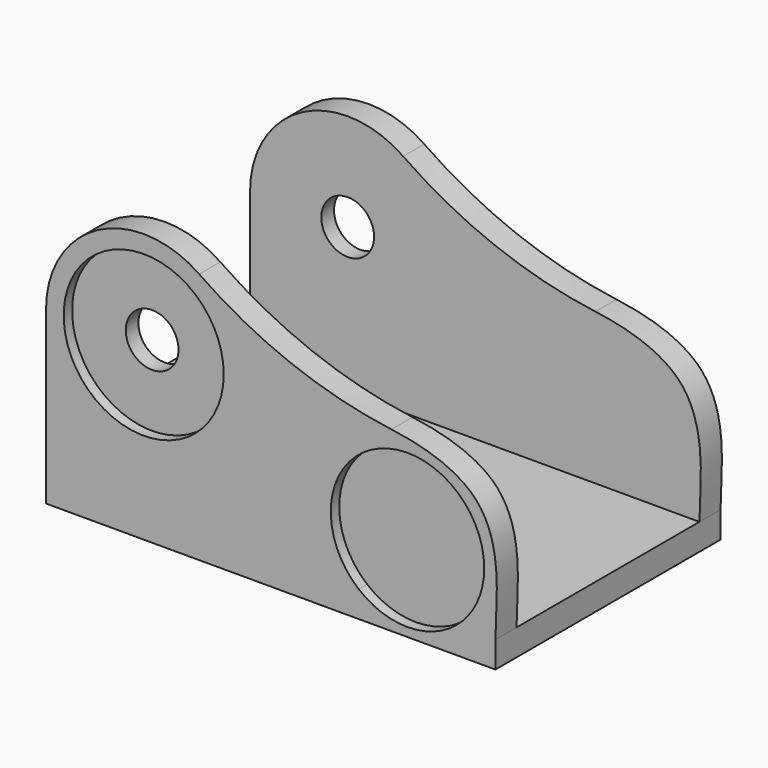
from build123d import *

# Parameters (mm, degrees)
F0_R            = 9.1
F0_W            = 2
F0_H            = 4
F0_R_2          = 3
F1_DEPTH        = 3
F1_COPIES_COUNT = 2
F1_COPIES_PITCH = 29
F2_DEPTH        = 32
F3_R            = 9.1
F4_DEPTH        = 3
F5_DEPTH        = 1.2
F3_R_2          = 3
F6_DEPTH        = 1.2


# Not quite as in the source:
# - a pattern or mirror of a feature is missing from the dataset's text; its kind, count and spacing are read off the source's solid


with BuildPart() as f1:
    # F0 (on Front) → F1 (new body)
    with BuildSketch(Plane.XZ):
        with BuildLine():
            Line((46.6587768439, 3), (51.1, 3))
            add(Edge.make_bspline(
                [(39.2721801194, 20.2002895195), (43.2600263156, 19.672514392), (52.7768717224, 16.5297183629), (51.1, 6.6124380804), (51.1, 3)],
                knots=[0.3415991708, 0.3415991708, 0.3415991708, 0.3415991708, 0.5830024084, 1, 1, 1, 1], degree=3))
            ThreePointArc((39.2721801194, 20.2002895195), (27.8400722418, 23.1174494268), (17.4097910893, 28.6321704107))
            ThreePointArc((17.4097910893, 28.6321704107), (5.9438716604, 29.329768082), (0, 19.5))
            Line((0, 19.5), (0, 7))
            Line((0, 7), (2, 7))
            Line((2, 7), (2, 3))
            Line((2, 3), (35.5412231561, 3))
            ThreePointArc((35.5412231561, 3), (37.3834628323, 17.6188568825), (49.825, 9.725))
            ThreePointArc((49.825, 9.725), (48.9938568825, 6.0084628323), (46.6587768439, 3))
        make_face()
        with Locations((11.1, 19.5)):
            Circle(F0_R, mode=Mode.SUBTRACT)
        with Locations((1, 5)):
            Rectangle(F0_W, F0_H)
        with BuildLine():
            Line((0, 3), (0, 0))
            Line((0, 0), (51.1, 0))
            Line((51.1, 0), (51.1, 3))
            Line((51.1, 3), (46.6587768439, 3))
            ThreePointArc((46.6587768439, 3), (41.1, 1), (35.5412231561, 3))
            Line((35.5412231561, 3), (2, 3))
            Line((2, 3), (0, 3))
        make_face()
        with BuildLine():
            Line((35.5412231561, 3), (46.6587768439, 3))
            ThreePointArc((46.6587768439, 3), (48.9938568825, 6.0084628323), (49.825, 9.725))
            ThreePointArc((49.825, 9.725), (37.3834628323, 17.6188568825), (35.5412231561, 3))
        make_face()
        with BuildLine():
            ThreePointArc((35.5412231561, 3), (41.1, 1), (46.6587768439, 3))
            Line((46.6587768439, 3), (35.5412231561, 3))
        make_face()
        with Locations((11.1, 19.5)):
            Circle(F0_R)
        with Locations((11.1, 19.5)):
            Circle(F0_R_2, mode=Mode.SUBTRACT)
    extrude(amount=-F1_DEPTH)


with BuildPart() as f1_copies_1:
    # F1_copies: instance of F1
    add(f1.part.moved(Location(Vector(0, 1, 0) * (1 * F1_COPIES_PITCH))))


with BuildPart() as f1_1:
    add(f1.part)

    add(f1_copies_1.part)  # F2 merges F1_copies_1
    # F0 (on Front) → F2 (join)
    with BuildSketch(Plane.XZ):
        with BuildLine():
            ThreePointArc((35.5412231561, 3), (41.1, 1), (46.6587768439, 3))
            Line((46.6587768439, 3), (35.5412231561, 3))
        make_face()
        with BuildLine():
            Line((0, 3), (0, 0))
            Line((0, 0), (51.1, 0))
            Line((51.1, 0), (51.1, 3))
            Line((51.1, 3), (46.6587768439, 3))
            ThreePointArc((46.6587768439, 3), (41.1, 1), (35.5412231561, 3))
            Line((35.5412231561, 3), (2, 3))
            Line((2, 3), (0, 3))
        make_face()
        with Locations((1, 5)):
            Rectangle(F0_W, F0_H)
    extrude(amount=-F2_DEPTH)

    # F3 (on face) → F4 (join)
    with BuildSketch(Plane(origin=(0, 32, 0), x_dir=(-1, 0, 0), z_dir=(0, 1, 0))):
        with BuildLine():
            Line((-35.5412231561, 3), (-2, 3))
            Line((-2, 3), (-2, 7))
            Line((-2, 7), (0, 7))
            Line((0, 7), (0, 19.5))
            ThreePointArc((0, 19.5), (-5.9438716604, 29.329768082), (-17.4097910893, 28.6321704107))
            ThreePointArc((-17.4097910893, 28.6321704107), (-24.6422981145, 24.4802718869), (-32.4642883797, 21.5882332434))
            ThreePointArc((-32.4642883797, 21.5882332434), (-35.8440967329, 20.7758663792), (-39.2721801194, 20.2002895195))
            add(Edge.make_bspline(
                [(-39.2721801194, 20.2002895195), (-43.2600263156, 19.672514392), (-50.5817963384, 17.2546092175), (-51.2780387876, 10.8269071453), (-51.2543959351, 7.7483589961)],
                knots=[0.3415991708, 0.3415991708, 0.3415991708, 0.3415991708, 0.5830024084, 0.8481388116, 0.8481388116, 0.8481388116, 0.8481388116], degree=3))
            add(Edge.make_bspline(
                [(-51.1, 3), (-50.9854700291, 4.1577635436), (-50.9621826453, 5.7020696678), (-51.1914335387, 7.3646437275), (-51.2543959351, 7.7483589961)],
                knots=[0, 0, 0, 0, 3.6124380804, 4.6797314617, 4.6797314617, 4.6797314617, 4.6797314617], degree=3))
            Line((-51.1, 3), (-46.6587768439, 3))
            ThreePointArc((-46.6587768439, 3), (-41.1, 18.45), (-35.5412231561, 3))
        make_face()
        with Locations((-11.1, 19.5)):
            Circle(F3_R, mode=Mode.SUBTRACT)
        with BuildLine():
            Line((-46.6587768439, 3), (-35.5412231561, 3))
            ThreePointArc((-35.5412231561, 3), (-41.1, 18.45), (-46.6587768439, 3))
        make_face()
    extrude(amount=-F4_DEPTH)

    # F0 (on Front) → F5 (cut)
    with BuildSketch(Plane.XZ):
        with Locations((11.1, 19.5)):
            Circle(F0_R)
        with Locations((11.1, 19.5)):
            Circle(F0_R_2, mode=Mode.SUBTRACT)
        with BuildLine():
            Line((35.5412231561, 3), (46.6587768439, 3))
            ThreePointArc((46.6587768439, 3), (48.9938568825, 6.0084628323), (49.825, 9.725))
            ThreePointArc((49.825, 9.725), (37.3834628323, 17.6188568825), (35.5412231561, 3))
        make_face()
        with BuildLine():
            ThreePointArc((35.5412231561, 3), (41.1, 1), (46.6587768439, 3))
            Line((46.6587768439, 3), (35.5412231561, 3))
        make_face()
    extrude(amount=-F5_DEPTH, mode=Mode.SUBTRACT)

    # F3 (on face) → F6 (cut)
    with BuildSketch(Plane(origin=(0, 32, 0), x_dir=(-1, 0, 0), z_dir=(0, 1, 0))):
        with Locations((-11.1, 19.5)):
            Circle(F3_R)
        with Locations((-11.1, 19.5)):
            Circle(F3_R_2, mode=Mode.SUBTRACT)
    extrude(amount=-F6_DEPTH, mode=Mode.SUBTRACT)


solid = f1_1.part
